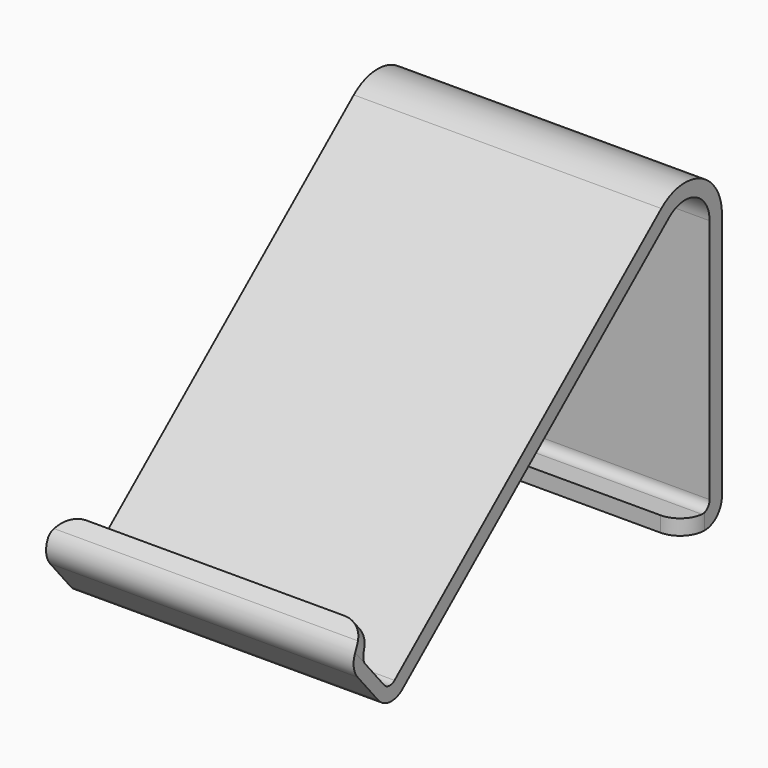
from build123d import *

# Parameters (mm, degrees)
F1_DEPTH = 50
F2_R     = 7
F3_R     = 3
F4_R     = 7.99999


# Not quite as in the source:
# - a fillet or chamfer is up to 0.001 mm smaller than in the source, because OpenCascade refuses the exact size


with BuildPart() as f1:
    # F0 (on Right) → F1 (new body, symmetric)
    with BuildSketch(Plane.YZ):
        with BuildLine():
            Line((-152.5870774385, 20.6831999642), (-135.231811977, 0))
            Line((-135.231811977, 0), (-21.4278760969, 95.4928406235))
            ThreePointArc((-21.4278760969, 95.4928406235), (-10.7738173826, 96.8954740627), (-5, 87.8323961924))
            Line((-5, 87.8323961924), (-5, 5))
            Line((-5, 5), (-15, 5))
            Line((-15, 5), (-15, 0))
            Line((-15, 0), (0, 0))
            Line((0, 0), (0, 87.8323961924))
            ThreePointArc((0, 87.8323961924), (-8.6607260739, 101.4270129979), (-24.6418141453, 99.3230628391))
            Line((-24.6418141453, 99.3230628391), (-135.381572253, 6.4013726543))
            Line((-135.381572253, 6.4013726543), (-146.9517492273, 20.1901726305))
            Line((-146.9517492273, 20.1901726305), (-140.8233936824, 25.332473508))
            Line((-140.8233936824, 25.332473508), (-143.3945441211, 28.3966512805))
            Line((-143.3945441211, 28.3966512805), (-152.5870774385, 20.6831999642))
        make_face()
    extrude(amount=F1_DEPTH, both=True)

    # F2
    f2_edges = [f1.edges().sort_by_distance(p)[0] for p in [
        (0, -135.231812, 0),
        (0, -152.587077, 20.6832),
        (0, 0, 0),
    ]]
    fillet(f2_edges, radius=F2_R)

    # F3
    f3_edges = [f1.edges().sort_by_distance(p)[0] for p in [
        (0, -146.951749, 20.190173),
        (0, -135.381572, 6.401373),
        (0, -5, 5),
    ]]
    fillet(f3_edges, radius=F3_R)

    # F4 (radius 8 in the source; OpenCascade refuses exactly that, so slightly less here)
    f4_edges = [f1.edges().sort_by_distance(p)[0] for p in [
        (50, -142.108969, 26.864562),
        (-50, -142.108969, 26.864562),
        (50, -15, 2.5),
        (-50, -15, 2.5),
    ]]
    fillet(f4_edges, radius=F4_R)


solid = f1.part
